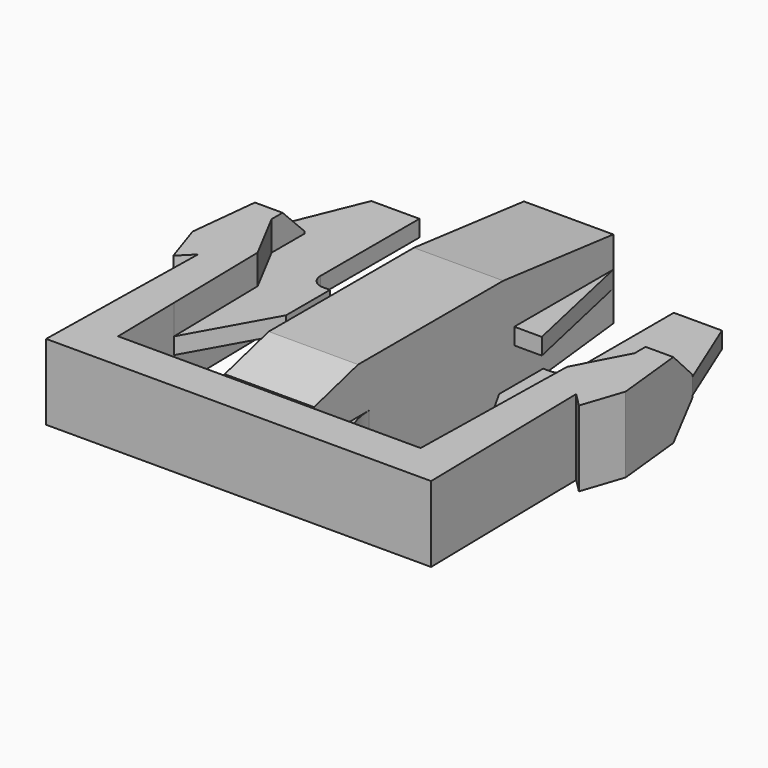
from build123d import *

# Parameters (mm, degrees)
F1_DEPTH    = 2.75
F2_DEPTH    = 0.6
F3_SIZE     = 2
F4_W        = 6.5
F4_H        = 27.2
F5_DEPTH    = 1.2
F6_C1_SIZE2 = 4
F6_C1_SIZE  = 1.1
F6_C2_SIZE2 = 1.1
F6_C2_SIZE  = 4
F7_C1_SIZE2 = 1.1
F7_C1_SIZE  = 10
F7_C2_SIZE2 = 10
F7_C2_SIZE  = 1.1


# Not quite as in the source:
# - a pattern or mirror of a feature is missing from the dataset's text; its kind, count and spacing are read off the source's solid


with BuildPart() as f1:
    # F0 (on Top) → F1 (new body, symmetric)
    with BuildSketch(Plane.XY):
        Polygon((3.25, 30), (0, 30), (-3.25, 30), (-3.25, 21), (-3.25, 7.8), (-3.25, 2.8), (-8.25, 2.8), (-11, 2.8), (-11.1000184963, 8), (-11.25, 15.7975959316), (-13.2, 19.5), (-13.2, 22.5), (-15, 22.5), (-15.75, 15.5), (-14.75, 12.5), (-13.75, 13.5), (-14, 0), (0, 0), (14, 0), (13.75, 13.5), (14.75, 12.5), (15.75, 15.5), (15, 22.5), (13.2, 22.5), (13.2, 19.5), (11.25, 15.7975959316), (11.1000184963, 8), (11, 2.8), (8.25, 2.8), (3.25, 2.8), (3.25, 7.8), (3.25, 21), align=None)
    extrude(amount=F1_DEPTH, both=True)

    # F0 (on Top) → F2 (join, symmetric)
    with BuildSketch(Plane.XY):
        with BuildLine():
            Line((-11.25, 15.7975959316), (-11.1000184963, 8))
            Line((-11.1000184963, 8), (-7.75, 14))
            Line((-7.75, 14), (-7.75, 18))
            Line((-7.75, 18), (-8.25, 18))
            ThreePointArc((-8.25, 18), (-8.9571067812, 18.2928932188), (-9.25, 19))
            Line((-9.25, 19), (-9.25, 28))
            Line((-9.25, 28), (-12.75, 28))
            Line((-12.75, 28), (-15, 22.5))
            Line((-15, 22.5), (-13.2, 22.5))
            Line((-13.2, 22.5), (-13.2, 19.5))
            Line((-13.2, 19.5), (-11.25, 15.7975959316))
        make_face()
        Polygon((-3.25, 21), (-3.25, 30), (-5.25, 21), align=None)
        Polygon((5.25, 21), (3.25, 30), (3.25, 21), align=None)
        with BuildLine():
            Line((7.75, 14), (11.1000184963, 8))
            Line((11.1000184963, 8), (11.25, 15.7975959316))
            Line((11.25, 15.7975959316), (13.2, 19.5))
            Line((13.2, 19.5), (13.2, 22.5))
            Line((13.2, 22.5), (15, 22.5))
            Line((15, 22.5), (12.75, 28))
            Line((12.75, 28), (9.25, 28))
            Line((9.25, 28), (9.25, 19))
            ThreePointArc((9.25, 19), (8.9571067812, 18.2928932188), (8.25, 18))
            Line((8.25, 18), (7.75, 18))
            Line((7.75, 18), (7.75, 14))
        make_face()
        with BuildLine():
            ThreePointArc((8.25, 2.8), (4.7144660941, 4.2644660941), (3.25, 7.8))
            Line((3.25, 7.8), (3.25, 2.8))
            Line((3.25, 2.8), (8.25, 2.8))
        make_face()
        with BuildLine():
            Line((-3.25, 2.8), (-3.25, 7.8))
            ThreePointArc((-3.25, 7.8), (-4.7144660941, 4.2644660941), (-8.25, 2.8))
            Line((-8.25, 2.8), (-3.25, 2.8))
        make_face()
    extrude(amount=F2_DEPTH, both=True)

    # F3
    f3_edges = [f1.edges().sort_by_distance(p)[0] for p in [
        (14.1, 22.5, 2.75),
        (14.1, 22.5, -2.75),
        (-14.1, 22.5, 2.75),
        (-14.1, 22.5, -2.75),
    ]]
    chamfer(f3_edges, length=F3_SIZE)

    # F4 (on face) → F5 (join)
    with BuildSketch(Plane.XY.offset(2.75)):
        with Locations((0, 16.4)):
            Rectangle(F4_W, F4_H)
    f5 = extrude(amount=F5_DEPTH)

    # F5_copies: F5 across plane
    add(f5.mirror(Plane(origin=(0, 0, 0), x_dir=(-1, 0, 0), z_dir=(0, 0, -1))))

    # F6: chamfer of 4 x 1.1 on 2 edges, made by hand

    # F6_c1
    f6_c1_edges = [f1.edges().sort_by_distance(p)[0] for p in [
        (0, 2.8, -3.95),
    ]]
    f6_c1_side = f1.faces().sort_by_distance((0, 2.8, -3.928))[0]
    chamfer(f6_c1_edges, length=F6_C1_SIZE, length2=F6_C1_SIZE2, reference=f6_c1_side)

    # F6_c2
    f6_c2_edges = [f1.edges().sort_by_distance(p)[0] for p in [
        (0, 2.8, 3.95),
    ]]
    f6_c2_side = f1.faces().sort_by_distance((0, 2.822, 3.95))[0]
    chamfer(f6_c2_edges, length=F6_C2_SIZE, length2=F6_C2_SIZE2, reference=f6_c2_side)

    # F7: chamfer of 1.1 x 10 on 2 edges, made by hand

    # F7_c1
    f7_c1_edges = [f1.edges().sort_by_distance(p)[0] for p in [
        (0, 30, 3.95),
    ]]
    f7_c1_side = f1.faces().sort_by_distance((0, 29.978, 3.95))[0]
    chamfer(f7_c1_edges, length=F7_C1_SIZE, length2=F7_C1_SIZE2, reference=f7_c1_side)

    # F7_c2
    f7_c2_edges = [f1.edges().sort_by_distance(p)[0] for p in [
        (0, 30, -3.95),
    ]]
    f7_c2_side = f1.faces().sort_by_distance((0, 30, -3.928))[0]
    chamfer(f7_c2_edges, length=F7_C2_SIZE, length2=F7_C2_SIZE2, reference=f7_c2_side)


solid = f1.part
